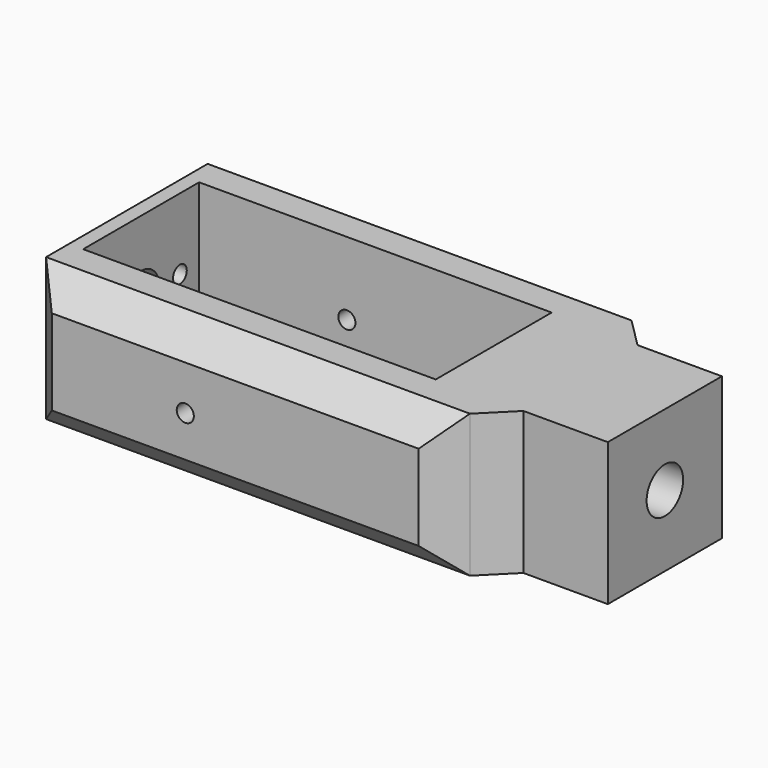
from build123d import *

# Parameters (mm, degrees)
F0_W      = 2.5
F0_H      = 24.4
F1_DEPTH  = 25
F4_R      = 1.5
F4_R_2    = 4
F5_DEPTH  = 2.5
F6_SIZE   = 5
F10_R     = 1.5
F11_DEPTH = 60
F8_W      = 25
F8_H      = 25
F12_DEPTH = 20
F13_SIZE  = 5.19999
F15_R     = 4
F16_DEPTH = 40


# Not quite as in the source:
# - a fillet or chamfer is up to 0.001 mm smaller than in the source, because OpenCascade refuses the exact size


with BuildPart() as f1:
    # F0 (on Top) → F1 (new body)
    with BuildSketch(Plane.XY):
        Polygon((-28.4, 12.2), (-25.9, 12.2), (-25.9, 12.7), (35.9, 12.7), (35.9, -12.7), (-25.9, -12.7), (-25.9, -12.2), (-28.4, -12.2), (-28.4, -22.7), (45.9, -22.7), (45.9, 22.7), (-28.4, 22.7), align=None)
        with Locations((-27.15, 0)):
            Rectangle(F0_W, F0_H)
    extrude(amount=F1_DEPTH)

    # F4 (on offset) → F5 (cut)
    with BuildSketch(Plane.YZ.offset(-28.4)):
        with Locations((-8.5, 12.5)):
            Circle(F4_R)
        with Locations((0, 12.5)):
            Circle(F4_R_2)
        with Locations((8.5, 12.5)):
            Circle(F4_R)
    extrude(amount=F5_DEPTH, mode=Mode.SUBTRACT)

    # F6
    f6_edges = [f1.edges().sort_by_distance(p)[0] for p in [
        (45.9, 22.7, 12.5),
        (-28.4, 22.7, 12.5),
        (8.75, 22.7, 0),
        (8.75, 22.7, 25),
        (-28.4, -22.7, 12.5),
        (45.9, -22.7, 12.5),
        (8.75, -22.7, 0),
        (8.75, -22.7, 25),
    ]]
    chamfer(f6_edges, length=F6_SIZE)

    # F10 (on offset) → F11 (cut)
    with BuildSketch(Plane.XZ.offset(22.7)):
        with Locations((0, 12.1945459396)):
            Circle(F10_R)
    extrude(amount=-F11_DEPTH, mode=Mode.SUBTRACT)

    # F8 (on offset) → F12 (join)
    with BuildSketch(Plane.YZ.offset(45.9)):
        with Locations((0, 12.5)):
            Rectangle(F8_W, F8_H)
    extrude(amount=F12_DEPTH)

    # F13 (size 5.2 in the source; OpenCascade refuses exactly that, so slightly less here)
    f13_edges = [f1.edges().sort_by_distance(p)[0] for p in [
        (45.9, 12.5, 12.5),
        (45.9, -12.5, 12.5),
    ]]
    chamfer(f13_edges, length=F13_SIZE)

    # F15 (on offset) → F16 (cut)
    with BuildSketch(Plane.YZ.offset(65.9)):
        with Locations((0, 12.5)):
            Circle(F15_R)
    extrude(amount=-F16_DEPTH, mode=Mode.SUBTRACT)


solid = f1.part
